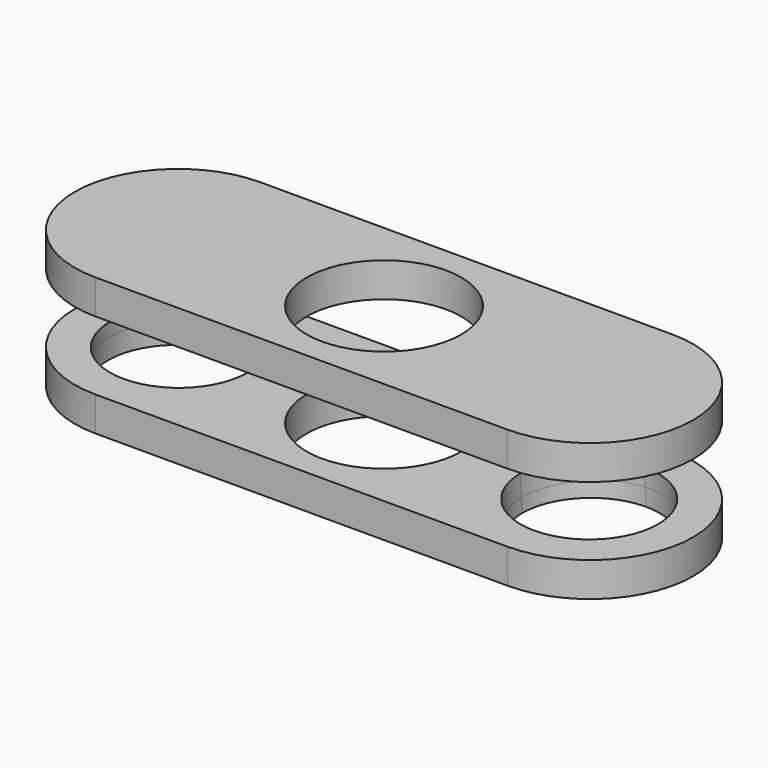
from build123d import *

# Parameters (mm, degrees)
F0_R     = 14.2875
F1_DEPTH = 3.175
F2_R     = 14.2875
F3_DEPTH = 3.175
F7_DEPTH = 19.05
F8_ANGLE = 3


# Not quite as in the source:
# - a feature names something its author has since deleted; it is built from what else it names


with BuildPart() as f1:
    # F0 (on Top) → F1 (new body, symmetric)
    with BuildSketch(Plane.XY):
        with BuildLine():
            ThreePointArc((38.1, -19.05), (57.15, 3e-10), (38.0999999995, 19.05))
            Line((38.0999999995, 19.05), (-38.1, 19.05))
            ThreePointArc((-38.1, 19.05), (-57.1499999995, -3e-10), (-38.0999999995, -19.05))
            Line((-38.0999999995, -19.05), (38.1, -19.05))
        make_face()
        Circle(F0_R, mode=Mode.SUBTRACT)
    extrude(amount=F1_DEPTH, both=True)


with BuildPart() as f3:
    # F2 (on Top) → F3 (new body, symmetric)
    with BuildSketch(Plane.XY):
        with BuildLine():
            ThreePointArc((38.1, -19.05), (57.15, 0), (38.1, 19.05))
            Line((38.1, 19.05), (-38.1, 19.05))
            Line((-38.1, 19.05), (-38.1, -19.05))
            Line((-38.1, -19.05), (38.1, -19.05))
        make_face()
        Circle(F2_R, mode=Mode.SUBTRACT)
        with BuildLine():
            Line((-38.1, -19.05), (-38.1, 19.05))
            ThreePointArc((-38.1, 19.05), (-57.15, 0), (-38.1, -19.05))
        make_face()
    extrude(amount=F3_DEPTH, both=True)


with BuildPart() as f1_1:
    # F5: moved
    add(f1.part.moved(Location((0, 0, 19.05))))


with BuildPart() as f7:
    # F6 (on Top) → F7 (new body, symmetric)
    with BuildSketch(Plane.XY):
        with BuildLine():
            Line((-38.1, -12.7), (-38.1, 12.7))
            ThreePointArc((-38.1, 12.7), (-50.8, 0), (-38.1, -12.7))
        make_face()
        with BuildLine():
            ThreePointArc((-38.1, -12.7), (-29.1197438789, -8.9802561211), (-25.4, 0))
            ThreePointArc((-25.4, 0), (-29.1197438789, 8.9802561211), (-38.1, 12.7))
            Line((-38.1, 12.7), (-38.1, -12.7))
        make_face()
    extrude(amount=F7_DEPTH, both=True)


with BuildPart() as f7_1:
    # F8: moved
    add(f7.part.rotate(Axis((-38.1, 0, 0), (0, 1, 0)), F8_ANGLE))


with BuildPart() as f9_1:
    # F9: instance of F7
    add(f7_1.part.mirror(Plane.YZ))


with BuildPart() as f1_2:
    add(f1_1.part)

    # F10: cut F7, F9_1
    add(f7_1.part, mode=Mode.SUBTRACT)
    add(f9_1.part, mode=Mode.SUBTRACT)


with BuildPart() as f3_1:
    add(f3.part)

    # F10: cut F7, F9_1
    add(f7_1.part, mode=Mode.SUBTRACT)
    add(f9_1.part, mode=Mode.SUBTRACT)


solid = Compound([f1_2.part, f3_1.part])
